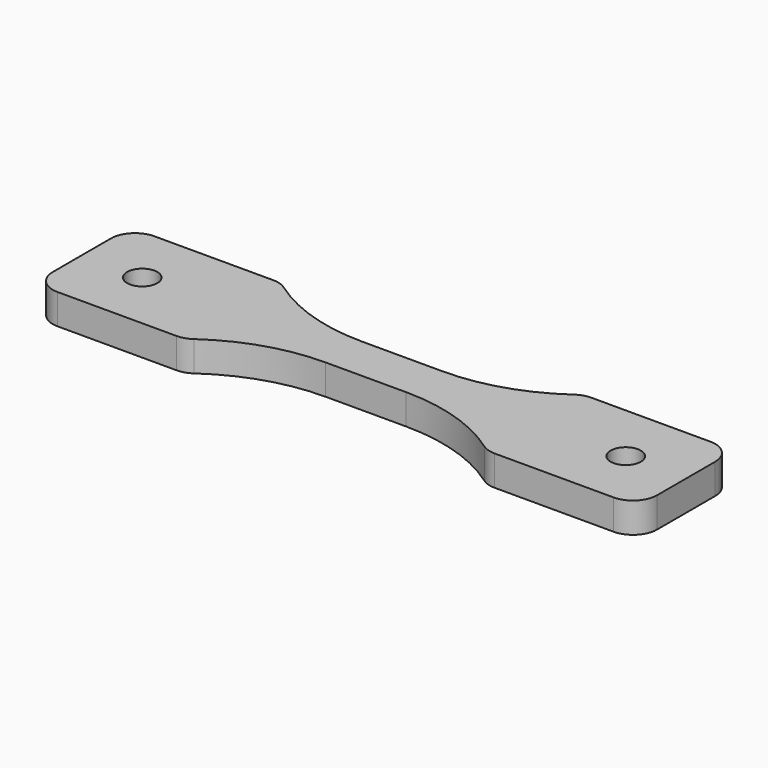
from build123d import *

# Parameters (mm, degrees)
F0_W        = 127
F0_H        = 25.4
F1_DEPTH    = 3.175
F2_W        = 63.5
F2_H        = 7.9375
F3_DEPTH    = 25.4
F4_T1_DEPTH = 6.35
F5_R        = 5.08
F6_R        = 3.175
F7_DEPTH    = 25.4


# Not quite as in the source:
# - a fillet or chamfer that OpenCascade refuses, or shapes differently, is made with other operations: its cross-section is extruded or revolved along the edge and cut away or added


with BuildPart() as f1:
    # F0 (on Top) → F1 (new body, symmetric)
    with BuildSketch(Plane.XY):
        Rectangle(F0_W, F0_H)
    extrude(amount=F1_DEPTH, both=True)

    # F2 (on face) → F3 (cut)
    with BuildSketch(Plane.XY.offset(3.175)):
        with Locations((0, 8.73125)):
            Rectangle(F2_W, F2_H)
        with Locations((0, -8.73125)):
            Rectangle(F2_W, F2_H)
    extrude(amount=-F3_DEPTH, mode=Mode.SUBTRACT)

    # F4: fillet of radius 38.1 on 4 edges, made by hand

    # F4_s2 → F4_t1 (join)
    with BuildSketch(Plane.XY.offset(-3.175)):
        with BuildLine():
            ThreePointArc((-31.75, 12.7), (-20.7694028252, 6.8014320042), (-8.4726807009, 4.7625))
            Line((-8.4726807009, 4.7625), (-31.75, 4.7625))
            Line((-31.75, 4.7625), (-31.75, 12.7))
        make_face()
        with BuildLine():
            ThreePointArc((8.4726807009, 4.7625), (20.7694028252, 6.8014320042), (31.75, 12.7))
            Line((31.75, 12.7), (31.75, 4.7625))
            Line((31.75, 4.7625), (8.4726807009, 4.7625))
        make_face()
        with BuildLine():
            ThreePointArc((31.75, -12.7), (20.7694028252, -6.8014320042), (8.4726807009, -4.7625))
            Line((8.4726807009, -4.7625), (31.75, -4.7625))
            Line((31.75, -4.7625), (31.75, -12.7))
        make_face()
        with BuildLine():
            ThreePointArc((-31.75, -12.7), (-20.7694028252, -6.8014320042), (-8.4726807009, -4.7625))
            Line((-8.4726807009, -4.7625), (-31.75, -4.7625))
            Line((-31.75, -4.7625), (-31.75, -12.7))
        make_face()
    extrude(amount=F4_T1_DEPTH)

    # F5
    f5_edges = [f1.edges().sort_by_distance(p)[0] for p in [
        (-63.5, 12.7, 0),
        (-31.75, 12.7, 0),
        (-63.5, -12.7, 0),
        (-31.75, -12.7, 0),
        (31.75, -12.7, 0),
        (63.5, -12.7, 0),
        (63.5, 12.7, 0),
        (31.75, 12.7, 0),
    ]]
    fillet(f5_edges, radius=F5_R)

    # F6 (on face) → F7 (cut)
    with BuildSketch(Plane.XY.offset(3.175)):
        with Locations((-50.8, 0)):
            Circle(F6_R)
        with Locations((50.8, 0)):
            Circle(F6_R)
    extrude(amount=-F7_DEPTH, mode=Mode.SUBTRACT)


solid = f1.part
